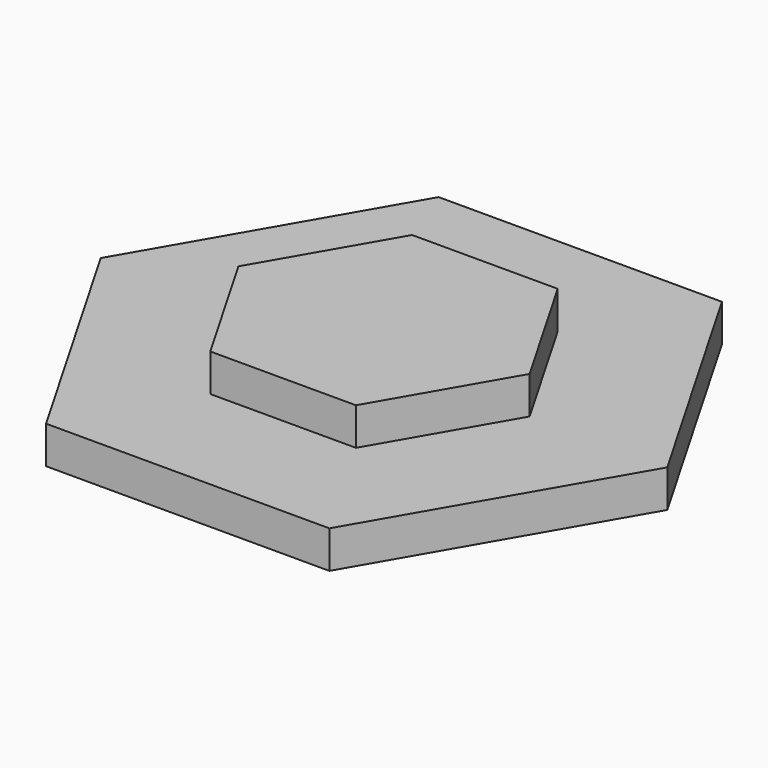
from build123d import *

# Parameters (mm, degrees)
F1_DEPTH = 2
F3_DEPTH = 2


# Not quite as in the source:
# - the program builds the solid bodies; features that only make, move or delete a surface that nothing else refers to are left out


with BuildPart() as f1:
    # F0 (on Top) → F1 (new body)
    with BuildSketch(Plane.XY):
        Polygon((7.5577008116, 13.0903217942), (-7.5577008116, 13.0903217942), (-15.1154016233, 0), (-7.5577008116, -13.0903217942), (7.5577008116, -13.0903217942), (15.1154016233, 0), align=None)
    extrude(amount=F1_DEPTH)

    # F2 (on face) → F3 (join)
    with BuildSketch(Plane.XY.offset(2)):
        Polygon((3.8847994902, 6.7286700942), (-3.8847994902, 6.7286700942), (-7.7695989803, 0), (-3.8847994902, -6.7286700942), (3.8847994902, -6.7286700942), (7.7695989803, 0), align=None)
    extrude(amount=F3_DEPTH)


solid = f1.part
